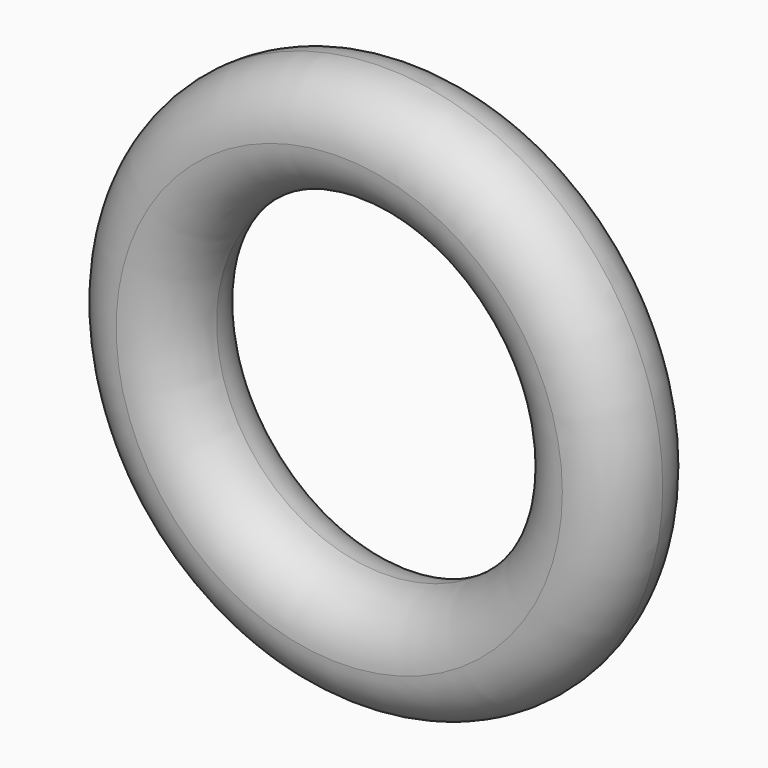
from build123d import *

# Parameters (mm, degrees)
F0_R     = 63.5
F0_R_2   = 38.1
F1_DEPTH = 25.4
F2_R     = 12.69999
F3_R     = 12.69999


# Not quite as in the source:
# - a fillet or chamfer is up to 0.001 mm smaller than in the source, because OpenCascade refuses the exact size


with BuildPart() as f1:
    # F0 (on Front) → F1 (new body)
    with BuildSketch(Plane.XZ):
        Circle(F0_R)
        Circle(F0_R_2, mode=Mode.SUBTRACT)
    extrude(amount=F1_DEPTH)

    # F2 (radius 12.7 in the source; OpenCascade refuses exactly that, so slightly less here)
    f2_edges = [f1.edges().sort_by_distance(p)[0] for p in [
        (-38.1, -25.4, 0),
        (-38.1, 0, 0),
    ]]
    fillet(f2_edges, radius=F2_R)

    # F3 (radius 12.7 in the source; OpenCascade refuses exactly that, so slightly less here)
    f3_edges = [f1.edges().sort_by_distance(p)[0] for p in [
        (-63.5, -25.4, 0),
        (-63.5, 0, 0),
    ]]
    fillet(f3_edges, radius=F3_R)


solid = f1.part
